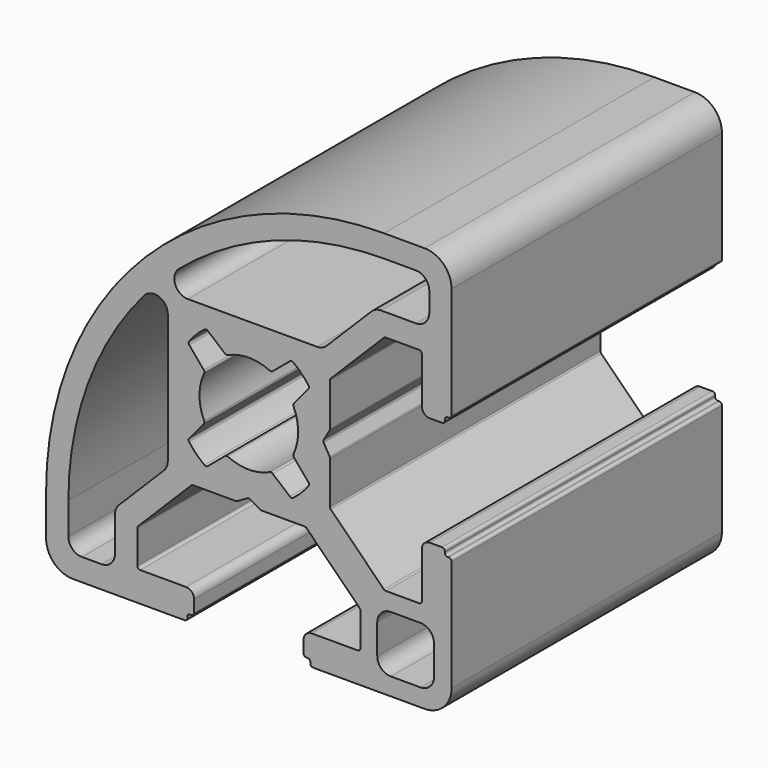
from build123d import *

# Parameters (mm, degrees)
F1_DEPTH = 25


# Not quite as in the source:
# - ends of sketch curves that miss each other by under 0.0002 mm in the source are joined


with BuildPart() as f1:
    # F0 (on Front) → F1 (new body)
    with BuildSketch(Plane.XZ):
        with BuildLine():
            ThreePointArc((-8.25, -10.132843), (-8.2347759065, -10.0563063135), (-8.1914213562, -9.9914216438))
            Line((-8.1914213562, -9.9914216438), (-4.263045, -6.063045))
            ThreePointArc((-4.263045, -6.063045), (-4.1981606865, -6.0196900935), (-4.121624, -6.004466))
            Line((-4.121624, -6.004466), (-0.95359, -6.004466))
            ThreePointArc((-0.95359, -6.004466), (-0.9018261715, -5.99765116), (-0.853589965, -5.9776710606))
            Line((-0.853589965, -5.9776710606), (-0.1, -5.542586))
            ThreePointArc((-0.1, -5.542586), (0, -5.515791), (0.100000035, -5.5425859394))
            Line((0.100000035, -5.5425859394), (0.85359, -5.977671))
            ThreePointArc((0.85359, -5.977671), (0.9018261715, -5.99765116), (0.95359, -6.004466))
            Line((0.95359, -6.004466), (4.121623, -6.004466))
            ThreePointArc((4.121623, -6.004466), (4.1981600131, -6.0196902288), (4.2630448562, -6.0630451438))
            Line((4.2630448562, -6.0630451438), (8.191421, -9.991421))
            ThreePointArc((8.191421, -9.991421), (8.2347757712, -10.0563059869), (8.25, -10.132843))
            Line((8.25, -10.132843), (8.25, -12.6))
            ThreePointArc((8.25, -12.6), (8.1914213562, -12.7414213562), (8.05, -12.8))
            Line((8.05, -12.8), (4.65, -12.8))
            ThreePointArc((4.65, -12.8), (4.2257359313, -12.9757359313), (4.05, -13.4))
            Line((4.05, -13.4), (4.05, -14.3))
            ThreePointArc((4.05, -14.3), (4.1085786438, -14.4414213562), (4.25, -14.5))
            Line((4.25, -14.5), (4.35, -14.5))
            ThreePointArc((4.35, -14.5), (4.4914213562, -14.5585786438), (4.55, -14.7))
            Line((4.55, -14.7), (4.55, -14.8))
            ThreePointArc((4.55, -14.8), (4.6085786438, -14.9414213562), (4.75, -15))
            Line((4.75, -15), (13, -15))
            ThreePointArc((13, -15), (14.4142135624, -14.4142135624), (15, -13))
            Line((15, -13), (15, -4.75))
            ThreePointArc((15, -4.75), (14.9414213562, -4.6085786438), (14.8, -4.55))
            Line((14.8, -4.55), (14.7, -4.55))
            ThreePointArc((14.7, -4.55), (14.5585786438, -4.4914213562), (14.5, -4.35))
            Line((14.5, -4.35), (14.5, -4.25))
            ThreePointArc((14.5, -4.25), (14.4414213562, -4.1085786438), (14.3, -4.05))
            Line((14.3, -4.05), (13.4, -4.05))
            ThreePointArc((13.4, -4.05), (12.9757359313, -4.2257359313), (12.8, -4.65))
            Line((12.8, -4.65), (12.8, -8.05))
            ThreePointArc((12.8, -8.05), (12.7414213562, -8.1914213562), (12.6, -8.25))
            Line((12.6, -8.25), (10.132843, -8.25))
            ThreePointArc((10.132843, -8.25), (10.0563063135, -8.2347759065), (9.9914216438, -8.1914213562))
            Line((9.9914216438, -8.1914213562), (6.063045, -4.263045))
            ThreePointArc((6.063045, -4.263045), (6.0196900935, -4.1981606865), (6.004466, -4.121624))
            Line((6.004466, -4.121624), (6.004466, -0.95359))
            ThreePointArc((6.004466, -0.95359), (5.99765116, -0.9018261715), (5.9776710606, -0.853589965))
            Line((5.9776710606, -0.853589965), (5.542586, -0.1))
            ThreePointArc((5.542586, -0.1), (5.515791, 0), (5.5425859394, 0.100000035))
            Line((5.5425859394, 0.100000035), (5.977671, 0.85359))
            ThreePointArc((5.977671, 0.85359), (5.99765116, 0.9018261715), (6.004466, 0.95359))
            Line((6.004466, 0.95359), (6.004466, 4.121623))
            ThreePointArc((6.004466, 4.121623), (6.0196902288, 4.1981600131), (6.0630451438, 4.2630448562))
            Line((6.0630451438, 4.2630448562), (9.991421, 8.191421))
            ThreePointArc((9.991421, 8.191421), (10.0563059869, 8.2347757712), (10.132843, 8.25))
            Line((10.132843, 8.25), (12.6, 8.25))
            ThreePointArc((12.6, 8.25), (12.7414213562, 8.1914213562), (12.8, 8.05))
            Line((12.8, 8.05), (12.8, 4.65))
            ThreePointArc((12.8, 4.65), (12.9757359313, 4.2257359313), (13.4, 4.05))
            Line((13.4, 4.05), (14.3, 4.05))
            ThreePointArc((14.3, 4.05), (14.4414213562, 4.1085786438), (14.5, 4.25))
            Line((14.5, 4.25), (14.5, 4.35))
            ThreePointArc((14.5, 4.35), (14.5585786438, 4.4914213562), (14.7, 4.55))
            Line((14.7, 4.55), (14.8, 4.55))
            ThreePointArc((14.8, 4.55), (14.9414213562, 4.6085786438), (15, 4.75))
            Line((15, 4.75), (15, 13))
            ThreePointArc((15, 13), (14.4142135624, 14.4142135624), (13, 15))
            Line((13, 15), (10, 15))
            ThreePointArc((10, 15), (-7.6776695297, 7.6776695297), (-15, -10))
            Line((-15, -10), (-15, -13))
            ThreePointArc((-15, -13), (-14.4142135624, -14.4142135624), (-13, -15))
            Line((-13, -15), (-4.75, -15))
            ThreePointArc((-4.75, -15), (-4.6085786438, -14.9414213562), (-4.55, -14.8))
            Line((-4.55, -14.8), (-4.55, -14.7))
            ThreePointArc((-4.55, -14.7), (-4.4914213562, -14.5585786438), (-4.35, -14.5))
            Line((-4.35, -14.5), (-4.25, -14.5))
            ThreePointArc((-4.25, -14.5), (-4.1085786438, -14.4414213562), (-4.05, -14.3))
            Line((-4.05, -14.3), (-4.05, -13.4))
            ThreePointArc((-4.05, -13.4), (-4.2257359313, -12.9757359313), (-4.65, -12.8))
            Line((-4.65, -12.8), (-8.05, -12.8))
            ThreePointArc((-8.05, -12.8), (-8.1914213562, -12.7414213562), (-8.25, -12.6))
            Line((-8.25, -12.6), (-8.25, -10.132843))
        make_face()
        with BuildLine():
            ThreePointArc((-13.35, -10), (-11.9068957969, -1.9185139644), (-7.7559600391, 5.1640490334))
            ThreePointArc((-7.7559600391, 5.1640490334), (-6.6494316246, 5.4528217522), (-5.995534, 4.514625))
            Line((-5.995534, 4.514625), (-5.995534, -5.047868))
            ThreePointArc((-5.995534, -5.047868), (-6.0716544675, -5.4305514324), (-6.2884272188, -5.7549747812))
            Line((-6.2884272188, -5.7549747812), (-9.607107, -9.073654))
            ThreePointArc((-9.607107, -9.073654), (-9.8238795325, -9.3980775676), (-9.9, -9.780761))
            Line((-9.9, -9.780761), (-9.9, -12.35))
            ThreePointArc((-9.9, -12.35), (-10.1928932188, -13.0571067812), (-10.9, -13.35))
            Line((-10.9, -13.35), (-12.35, -13.35))
            ThreePointArc((-12.35, -13.35), (-13.0571067812, -13.0571067812), (-13.35, -12.35))
            Line((-13.35, -12.35), (-13.35, -10))
        make_face(mode=Mode.SUBTRACT)
        with BuildLine():
            Line((10.5, -9.5), (12.7, -9.5))
            ThreePointArc((12.7, -9.5), (13.4071067812, -9.7928932188), (13.7, -10.5))
            Line((13.7, -10.5), (13.7, -12.7))
            ThreePointArc((13.7, -12.7), (13.4071067812, -13.4071067812), (12.7, -13.7))
            Line((12.7, -13.7), (10.5, -13.7))
            ThreePointArc((10.5, -13.7), (9.7928932188, -13.4071067812), (9.5, -12.7))
            Line((9.5, -12.7), (9.5, -10.5))
            ThreePointArc((9.5, -10.5), (9.7928932188, -9.7928932188), (10.5, -9.5))
        make_face(mode=Mode.SUBTRACT)
        with BuildLine():
            ThreePointArc((3.0353602524, 4.4052226992), (3.1580769226, 4.4519286863), (3.2833112184, 4.4124672935))
            ThreePointArc((3.2833112184, 4.4124672935), (3.8890875076, 3.8890870855), (4.4124676372, 3.2833107301))
            ThreePointArc((4.4124676372, 3.2833107301), (4.4519286776, 3.1580766242), (4.4052226992, 3.0353602524))
            Line((4.4052226992, 3.0353602524), (3.334407, 1.759212))
            ThreePointArc((3.334407, 1.759212), (3.2893137224, 1.6566579747), (3.3064409894, 1.545944995))
            ThreePointArc((3.3064409894, 1.545944995), (3.65, 0), (3.3064412445, -1.5459451143))
            ThreePointArc((3.3064412445, -1.5459451143), (3.2893137224, -1.6566579747), (3.3344073008, -1.7592117476))
            Line((3.3344073008, -1.7592117476), (4.405223, -3.03536))
            ThreePointArc((4.405223, -3.03536), (4.4519286863, -3.1580769226), (4.4124672935, -3.2833112184))
            ThreePointArc((4.4124672935, -3.2833112184), (3.8890870855, -3.8890875076), (3.2833107301, -4.4124676372))
            ThreePointArc((3.2833107301, -4.4124676372), (3.1580766242, -4.4519286776), (3.0353602524, -4.4052226992))
            Line((3.0353602524, -4.4052226992), (1.759212, -3.334407))
            ThreePointArc((1.759212, -3.334407), (1.6566579747, -3.2893137224), (1.545944995, -3.3064409894))
            ThreePointArc((1.545944995, -3.3064409894), (0, -3.65), (-1.5459451143, -3.3064412445))
            ThreePointArc((-1.5459451143, -3.3064412445), (-1.6566579747, -3.2893137224), (-1.7592117476, -3.3344073008))
            Line((-1.7592117476, -3.3344073008), (-3.03536, -4.405223))
            ThreePointArc((-3.03536, -4.405223), (-3.1580769226, -4.4519286863), (-3.2833112184, -4.4124672935))
            ThreePointArc((-3.2833112184, -4.4124672935), (-3.8890875076, -3.8890870855), (-4.4124676372, -3.2833107301))
            ThreePointArc((-4.4124676372, -3.2833107301), (-4.4519286776, -3.1580766242), (-4.4052226992, -3.0353602524))
            Line((-4.4052226992, -3.0353602524), (-3.334407, -1.759212))
            ThreePointArc((-3.334407, -1.759212), (-3.2893137224, -1.6566579747), (-3.3064409894, -1.545944995))
            ThreePointArc((-3.3064409894, -1.545944995), (-3.65, 0), (-3.3064412445, 1.5459451143))
            ThreePointArc((-3.3064412445, 1.5459451143), (-3.2893137224, 1.6566579747), (-3.3344073008, 1.7592117476))
            Line((-3.3344073008, 1.7592117476), (-4.405223, 3.03536))
            ThreePointArc((-4.405223, 3.03536), (-4.4519286863, 3.1580769226), (-4.4124672935, 3.2833112184))
            ThreePointArc((-4.4124672935, 3.2833112184), (-3.8890870855, 3.8890875076), (-3.2833107301, 4.4124676372))
            ThreePointArc((-3.2833107301, 4.4124676372), (-3.1580766242, 4.4519286776), (-3.0353602524, 4.4052226992))
            Line((-3.0353602524, 4.4052226992), (-1.759212, 3.334407))
            ThreePointArc((-1.759212, 3.334407), (-1.6566579747, 3.2893137224), (-1.545944995, 3.3064409894))
            ThreePointArc((-1.545944995, 3.3064409894), (0, 3.65), (1.5459451143, 3.3064412445))
            ThreePointArc((1.5459451143, 3.3064412445), (1.6566579747, 3.2893137224), (1.7592117476, 3.3344073008))
            Line((1.7592117476, 3.3344073008), (3.0353602524, 4.4052226992))
        make_face(mode=Mode.SUBTRACT)
        with BuildLine():
            ThreePointArc((-4.514625, 5.995534), (-5.4528210376, 6.6494323984), (-5.1640477551, 7.7559607133))
            ThreePointArc((-5.1640477551, 7.7559607133), (1.9185146258, 11.9068960409), (10, 13.35))
            Line((10, 13.35), (12.35, 13.35))
            ThreePointArc((12.35, 13.35), (13.0571067812, 13.0571067812), (13.35, 12.35))
            Line((13.35, 12.35), (13.35, 10.9))
            ThreePointArc((13.35, 10.9), (13.0571067812, 10.1928932188), (12.35, 9.9))
            Line((12.35, 9.9), (9.780761, 9.9))
            ThreePointArc((9.780761, 9.9), (9.3980778943, 9.8238796678), (9.0736547188, 9.6071072812))
            Line((9.0736547188, 9.6071072812), (5.754975, 6.288427))
            ThreePointArc((5.754975, 6.288427), (5.4305514324, 6.0716544675), (5.047868, 5.995534))
            Line((5.047868, 5.995534), (-4.514625, 5.995534))
        make_face(mode=Mode.SUBTRACT)
    extrude(amount=F1_DEPTH)


solid = f1.part
